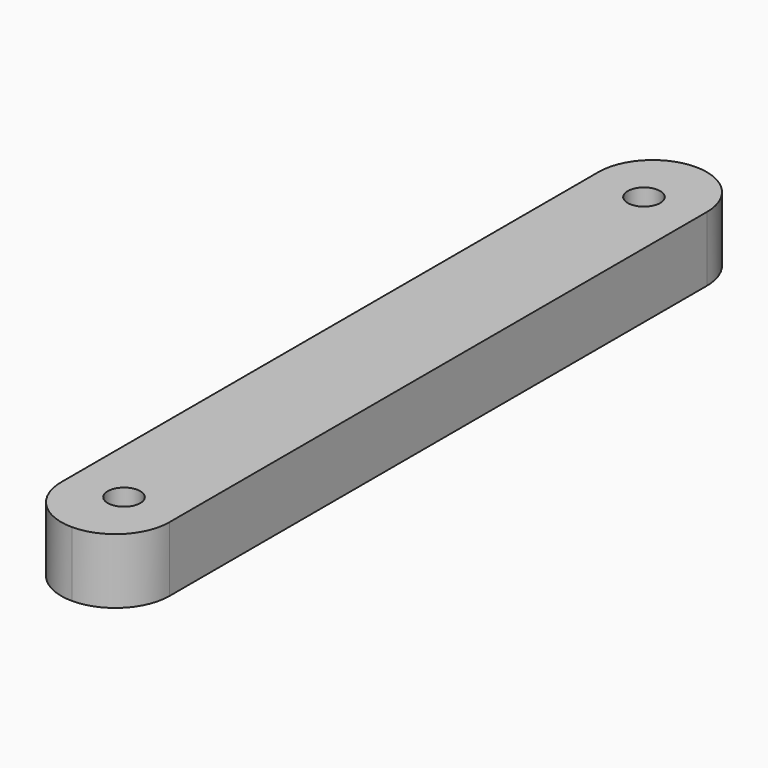
from build123d import *

# Parameters (mm, degrees)
F0_W     = 254
F0_H     = 152.4
F1_DEPTH = 914.4
F3_D     = 76.2
F4_R     = 126.99999


# Not quite as in the source:
# - a fillet or chamfer is up to 0.001 mm smaller than in the source, because OpenCascade refuses the exact size


with BuildPart() as f1:
    # F0 (on Front) → F1 (new body, symmetric)
    with BuildSketch(Plane.XZ):
        Rectangle(F0_W, F0_H)
    extrude(amount=F1_DEPTH, both=True)

    # F3 (through all)
    with Locations(Plane.XY.offset(76.2)):
        with Locations((0, 762), (0, -762)):
            Hole(F3_D / 2)

    # F4 (radius 127 in the source; OpenCascade refuses exactly that, so slightly less here)
    f4_edges = [f1.edges().sort_by_distance(p)[0] for p in [
        (127, -914.4, 0),
        (-127, -914.4, 0),
        (127, 914.4, 0),
        (-127, 914.4, 0),
    ]]
    fillet(f4_edges, radius=F4_R)


solid = f1.part
